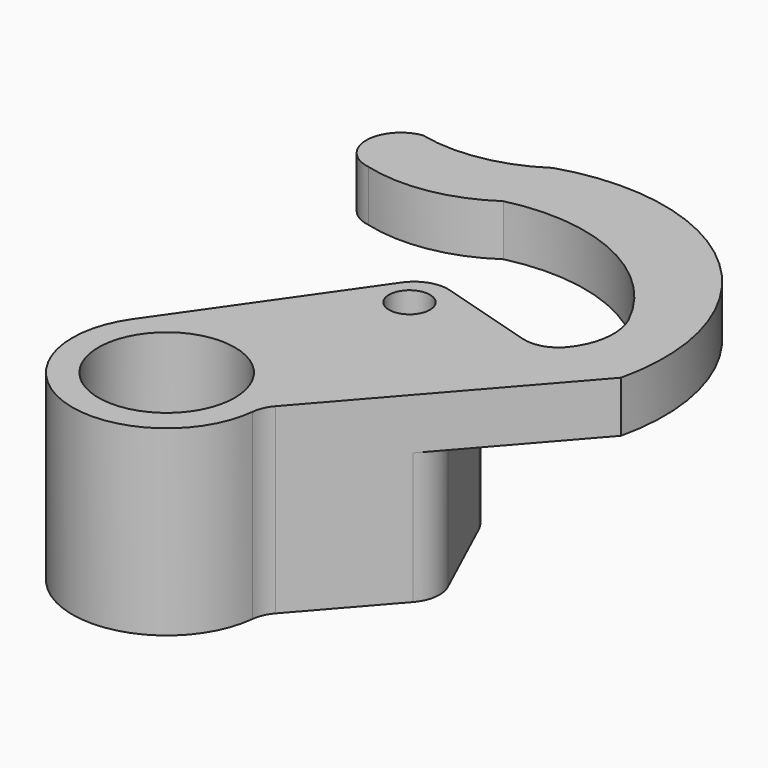
from build123d import *

# Parameters (mm, degrees)
F0_R        = 2
F0_R_2      = 0.6
F1_DEPTH    = 5.35
F2_DEPTH    = 3.85
F3_T1_DEPTH = 1.5
F3_T3_DEPTH = 5.35
F3_T5_DEPTH = 8.9622341314
F3_T7_DEPTH = 4.9810546268
F3_T9_DEPTH = 5.470707469


# Not quite as in the source:
# - a fillet or chamfer that OpenCascade refuses, or shapes differently, is made with other operations: its cross-section is extruded or revolved along the edge and cut away or added


with BuildPart() as f1:
    # F0 (on Top) → F1 (new body)
    with BuildSketch(Plane.XY):
        with BuildLine():
            ThreePointArc((-2.2671417814, 1.5828117838), (-0.8296318384, -2.637600427), (2.765, 0))
            Line((2.765, 0), (5.5232667008, 3.1497960053))
            Line((5.5232667008, 3.1497960053), (3.8210715694, 6.8505014831))
            Line((3.8210715694, 6.8505014831), (1.8260751385, 7.4457344599))
            Line((1.8260751385, 7.4457344599), (-2.2671417814, 1.5828117838))
        make_face()
        Circle(F0_R, mode=Mode.SUBTRACT)
        with Locations((2.165, 6.195)):
            Circle(F0_R_2, mode=Mode.SUBTRACT)
        with BuildLine():
            Line((3.8210715694, 6.8505014831), (5.5232667008, 3.1497960053))
            Line((5.5232667008, 3.1497960053), (8.2815334016, 6.2995920106))
            ThreePointArc((8.2815334016, 6.2995920106), (6.5094775109, 12.1209007662), (0.5720401491, 13.4530626491))
            ThreePointArc((0.5720401491, 13.4530626491), (-1.0341388497, 12.8062514702), (-2.765, 12.8541613445))
            ThreePointArc((-2.765, 12.8541613445), (-3.6292192652, 11.8541613445), (-2.765, 10.8541613445))
            ThreePointArc((-2.765, 10.8541613445), (-0.9627220535, 10.7761212346), (0.7094162112, 11.4530626491))
            ThreePointArc((0.7094162112, 11.4530626491), (4.1711880344, 11.0946407177), (6.6333355769, 8.6349334352))
            ThreePointArc((6.6333355769, 8.6349334352), (6.6911609557, 7.2849011256), (5.8160680002, 6.2552685064))
            Line((5.8160680002, 6.2552685064), (3.8210715694, 6.8505014831))
        make_face()
    extrude(amount=F1_DEPTH)

    # F0 (on Top) → F2 (cut)
    with BuildSketch(Plane.XY):
        with BuildLine():
            Line((3.8210715694, 6.8505014831), (5.5232667008, 3.1497960053))
            Line((5.5232667008, 3.1497960053), (8.2815334016, 6.2995920106))
            ThreePointArc((8.2815334016, 6.2995920106), (6.5094775109, 12.1209007662), (0.5720401491, 13.4530626491))
            ThreePointArc((0.5720401491, 13.4530626491), (-1.0341388497, 12.8062514702), (-2.765, 12.8541613445))
            ThreePointArc((-2.765, 12.8541613445), (-3.6292192652, 11.8541613445), (-2.765, 10.8541613445))
            ThreePointArc((-2.765, 10.8541613445), (-0.9627220535, 10.7761212346), (0.7094162112, 11.4530626491))
            ThreePointArc((0.7094162112, 11.4530626491), (4.1711880344, 11.0946407177), (6.6333355769, 8.6349334352))
            ThreePointArc((6.6333355769, 8.6349334352), (6.6911609557, 7.2849011256), (5.8160680002, 6.2552685064))
            Line((5.8160680002, 6.2552685064), (3.8210715694, 6.8505014831))
        make_face()
    extrude(amount=F2_DEPTH, mode=Mode.SUBTRACT)

    # F3: fillet of radius 1 on 5 edges, made by hand

    # F3_s2 → F3_t1 (join)
    with BuildSketch(Plane.XY.offset(3.85)):
        with BuildLine():
            ThreePointArc((5.3238056204, 6.4021413514), (5.9123715372, 6.4072989523), (6.3960858458, 6.7426449035))
            ThreePointArc((6.3960858458, 6.7426449035), (6.1312771268, 6.4689663976), (5.8160680002, 6.2552685064))
            Line((5.8160680002, 6.2552685064), (5.3238056204, 6.4021413514))
        make_face()
    extrude(amount=F3_T1_DEPTH)

    # F3_s4 → F3_t3 (join)
    with BuildSketch(Plane.XY):
        with BuildLine():
            ThreePointArc((2.7493247705, -0.294003922), (2.8276858836, 0.0009129267), (2.9913388108, 0.258467059))
            Line((2.9913388108, 0.258467059), (2.765, 0))
            ThreePointArc((2.765, 0), (2.7610784116, -0.1472107494), (2.7493247705, -0.294003922))
        make_face()
    extrude(amount=F3_T3_DEPTH)

    # F3_s6 → F3_t5 (cut)
    with BuildSketch(Plane.XY.offset(-1.8061170657)):
        with BuildLine():
            ThreePointArc((1.41251371, 6.8533694021), (1.9030466902, 7.2251109605), (2.5183648424, 7.2391808767))
            Line((2.5183648424, 7.2391808767), (1.8260751385, 7.4457344599))
            Line((1.8260751385, 7.4457344599), (1.41251371, 6.8533694021))
        make_face()
    extrude(amount=F3_T5_DEPTH, mode=Mode.SUBTRACT)

    # F3_s8 → F3_t7 (cut)
    with BuildSketch(Plane.XY.offset(-1.1310546268)):
        with BuildLine():
            ThreePointArc((3.3875351793, 6.9798526699), (3.757108564, 6.7768067273), (4.010129337, 6.4394750953))
            Line((4.010129337, 6.4394750953), (3.8210715694, 6.8505014831))
            Line((3.8210715694, 6.8505014831), (3.3875351793, 6.9798526699))
        make_face()
    extrude(amount=F3_T7_DEPTH, mode=Mode.SUBTRACT)

    # F3_s10 → F3_t9 (cut)
    with BuildSketch(Plane.XY.offset(-1.620707469)):
        with BuildLine():
            ThreePointArc((5.2523626005, 3.738762728), (5.3335017603, 3.1773237272), (5.0961768875, 2.6620818233))
            Line((5.0961768875, 2.6620818233), (5.5232667008, 3.1497960053))
            Line((5.5232667008, 3.1497960053), (5.2523626005, 3.738762728))
        make_face()
    extrude(amount=F3_T9_DEPTH, mode=Mode.SUBTRACT)


solid = f1.part
